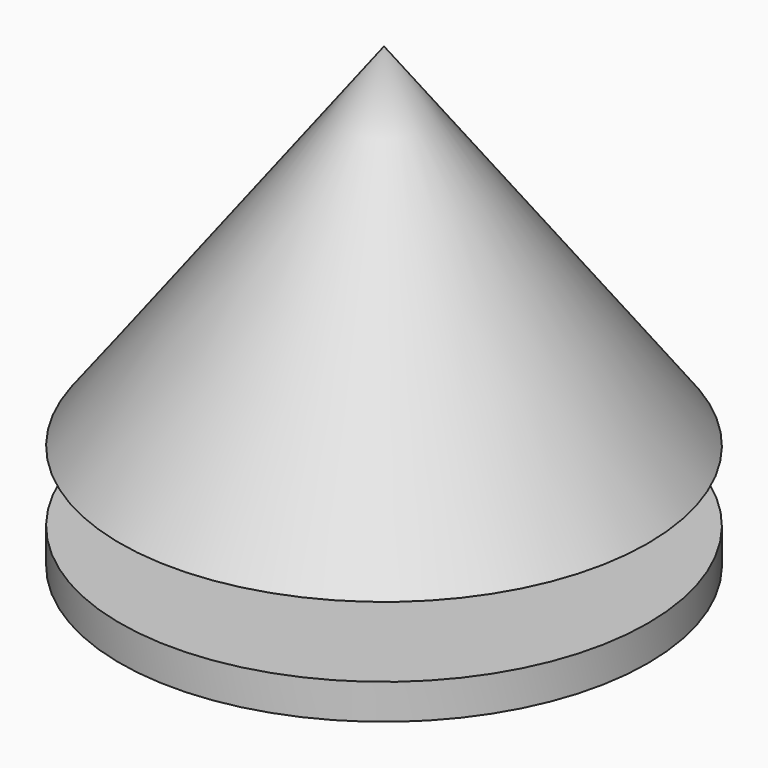
from build123d import *

# Parameters (mm, degrees)
F3_R     = 6.35
F4_DEPTH = 5.08
F5_R     = 19.05
F5_R_2   = 6.35
F6_DEPTH = 2.54
F7_R     = 5.08
F8_DEPTH = 19.05


with BuildPart() as f2:
    # F1 (on Front) → F2 (revolve)
    with BuildSketch(Plane.XZ):
        Polygon((0, 25.4), (0, 0), (19.05, 0), align=None)
    revolve(axis=Axis((0, 0, 12.7), (0, 0, 1)))

    # F3 (on face) → F4 (join)
    with BuildSketch(Plane.XY):
        Circle(F3_R)
    extrude(amount=-F4_DEPTH)

    # F5 (on face) → F6 (join)
    with BuildSketch(Plane(origin=(0, 0, -5.08), x_dir=(1, 0, 0), z_dir=(0, 0, -1))):
        Circle(F5_R)
        Circle(F5_R_2, mode=Mode.SUBTRACT)
        Circle(F5_R_2)
    extrude(amount=F6_DEPTH)

    # F7 (on face) → F8 (cut)
    with BuildSketch(Plane(origin=(0, 0, -7.62), x_dir=(1, 0, 0), z_dir=(0, 0, -1))):
        Circle(F7_R)
    extrude(amount=-F8_DEPTH, mode=Mode.SUBTRACT)


solid = f2.part
